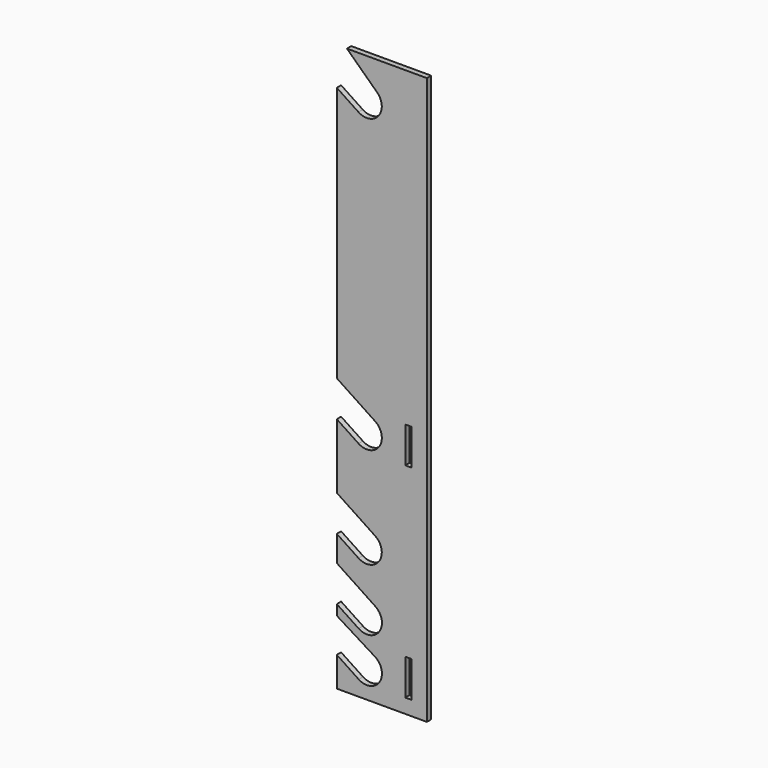
from build123d import *

# Parameters (mm, degrees)
F0_W     = 12.7
F0_H     = 76.2
F1_DEPTH = 11.43


# Not quite as in the source:
# - a feature names something its author has since deleted; it is built from what else it names


with BuildPart() as f1:
    # F0 (on Front) → F1 (new body)
    with BuildSketch(Plane.XZ):
        with BuildLine():
            Line((86.44143009, 487.5982903777), (-82.6555196025, 487.5982903777))
            Line((-82.6555196025, 487.5982903777), (-18.7736136836, 426.7721436688))
            ThreePointArc((-18.7736136836, 426.7721436688), (-15.8484759418, 383.977401572), (-58.2239000145, 377.323844885))
            Line((-58.2239000145, 377.323844885), (-104.05856991, 407.7417460511))
            Line((-104.05856991, 407.7417460511), (-104.05856991, -133.2205747848))
            Line((-104.05856991, -133.2205747848), (-23.008097061, -186.9833762889))
            ThreePointArc((-23.008097061, -186.9833762889), (-14.1002365767, -230.9921824712), (-58.109042759, -239.9000429556))
            Line((-58.109042759, -239.9000429556), (-104.05856991, -209.4205747848))
            Line((-104.05856991, -209.4205747848), (-104.05856991, -346.656112826))
            Line((-104.05856991, -346.656112826), (-23.121974943, -400.3433762889))
            ThreePointArc((-23.121974943, -400.3433762889), (-14.2141144586, -444.3521824712), (-58.2229206409, -453.2600429556))
            Line((-58.2229206409, -453.2600429556), (-104.05856991, -422.856112826))
            Line((-104.05856991, -422.856112826), (-104.05856991, -477.484384418))
            Line((-104.05856991, -477.484384418), (-22.7666009966, -531.4073762889))
            ThreePointArc((-22.7666009966, -531.4073762889), (-13.8587405122, -575.4161824712), (-57.8675466945, -584.3240429556))
            Line((-57.8675466945, -584.3240429556), (-104.05856991, -553.684384418))
            Line((-104.05856991, -553.684384418), (-104.05856991, -575.4260893394))
            Line((-104.05856991, -575.4260893394), (-23.5744710882, -625.3769093504))
            ThreePointArc((-23.5744710882, -625.3769093504), (-13.5964073743, -669.50213472), (-57.8674036509, -678.8121378395))
            Line((-57.8674036509, -678.8121378395), (-104.05856991, -648.172744022))
            Line((-104.05856991, -648.172744022), (-104.05856991, -711.2817096223))
            Line((-104.05856991, -711.2817096223), (47.07143009, -711.2817096223))
            Line((47.07143009, -711.2817096223), (86.44143009, -711.2817096223))
            Line((86.44143009, -711.2817096223), (86.44143009, 487.5982903777))
        make_face()
        with Locations((47.07143009, -642.7017096223)):
            Rectangle(F0_W, F0_H, mode=Mode.SUBTRACT)
        with Locations((47.07143009, -210.3231889248)):
            Rectangle(F0_W, F0_H, mode=Mode.SUBTRACT)
    extrude(amount=F1_DEPTH)


solid = f1.part
